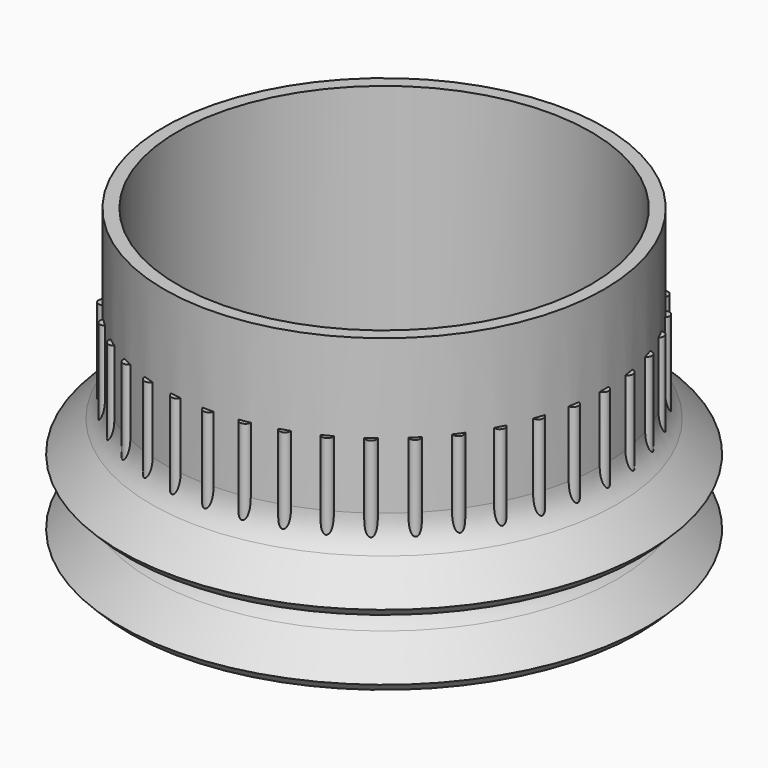
from build123d import *


with BuildPart() as f1:
    # F0 (on Front) → F1 (revolve)
    with BuildSketch(Plane.XZ):
        with BuildLine():
            Line((60, -14.1421356237), (52.9289321881, -7.0710678119))
            ThreePointArc((52.9289321881, -7.0710678119), (50.7612046749, -3.8268343237), (50, 0))
            Line((50, 0), (50, 5.8076118446))
            ThreePointArc((50, 5.8076118446), (50.4038059223, 5.9748737342), (50.8076118446, 5.8076118446))
            Line((50.8076118446, 5.8076118446), (57.8786796564, -1.2634559673))
            Line((57.8786796564, -1.2634559673), (60, 0.8578643763))
            Line((60, 0.8578643763), (52.9289321881, 7.9289321881))
            ThreePointArc((52.9289321881, 7.9289321881), (50.7612046749, 11.1731656763), (50, 15))
            Line((50, 15), (50, 47.5))
            Line((50, 47.5), (50, 50))
            Line((50, 50), (47, 50))
            Line((47, 50), (47, 0))
            ThreePointArc((47, 0), (47.9895660774, -4.9748846207), (50.8076118446, -9.1923881554))
            Line((50.8076118446, -9.1923881554), (57.8786796564, -16.2634559673))
            Line((57.8786796564, -16.2634559673), (60, -14.1421356237))
        make_face()
    revolve(axis=Axis((0, 0, 26.1525176466), (0, 0, 1)))

    # F3 (on offset) → F4 (join, up to the next surface of F1)
    with BuildSketch(Plane.XY.offset(30)):
        with BuildLine():
            ThreePointArc((-1.227725711, 49.9849246231), (0, 50), (1.227725711, 49.9849246231))
            ThreePointArc((1.227725711, 49.9849246231), (0, 51), (-1.227725711, 49.9849246231))
        make_face()
        with BuildLine():
            ThreePointArc((6.6067545733, 49.5615858706), (7.821723252, 49.3844170298), (9.0319753137, 49.177468641))
            ThreePointArc((9.0319753137, 49.177468641), (7.9781577171, 50.3721053704), (6.6067545733, 49.5615858706))
        make_face()
        with BuildLine():
            ThreePointArc((14.2785546334, 47.9178763885), (15.4508497187, 47.5528258148), (16.6138277088, 47.1591001702))
            ThreePointArc((16.6138277088, 47.1591001702), (15.7598667131, 48.5038823311), (14.2785546334, 47.9178763885))
        make_face()
        with BuildLine():
            ThreePointArc((21.5987692907, 45.0942697593), (22.699524987, 44.5503262094), (23.7865925275, 43.9795181412))
            ThreePointArc((23.7865925275, 43.9795181412), (23.1535154867, 45.4413327336), (21.5987692907, 45.0942697593))
        make_face()
        with BuildLine():
            ThreePointArc((28.3871505658, 41.1602925494), (29.3892626146, 40.4508497187), (30.373652495, 39.7170144159))
            ThreePointArc((30.373652495, 39.7170144159), (29.9770478669, 41.2598667131), (28.3871505658, 41.1602925494))
        make_face()
        with BuildLine():
            ThreePointArc((34.4765459824, 36.2128123338), (35.3553390593, 35.3553390593), (36.2128123338, 34.4765459824))
            ThreePointArc((36.2128123338, 34.4765459824), (36.0624458405, 36.0624458405), (34.4765459824, 36.2128123338))
        make_face()
        with BuildLine():
            ThreePointArc((39.7170144159, 30.373652495), (40.4508497187, 29.3892626146), (41.1602925494, 28.3871505658))
            ThreePointArc((41.1602925494, 28.3871505658), (41.2598667131, 29.9770478669), (39.7170144159, 30.373652495))
        make_face()
        with BuildLine():
            ThreePointArc((43.9795181412, 23.7865925275), (44.5503262094, 22.699524987), (45.0942697593, 21.5987692907))
            ThreePointArc((45.0942697593, 21.5987692907), (45.4413327336, 23.1535154867), (43.9795181412, 23.7865925275))
        make_face()
        with BuildLine():
            ThreePointArc((47.1591001702, 16.6138277088), (47.5528258148, 15.4508497187), (47.9178763885, 14.2785546334))
            ThreePointArc((47.9178763885, 14.2785546334), (48.5038823311, 15.7598667131), (47.1591001702, 16.6138277088))
        make_face()
        with BuildLine():
            ThreePointArc((49.177468641, 9.0319753137), (49.3844170298, 7.821723252), (49.5615858706, 6.6067545733))
            ThreePointArc((49.5615858706, 6.6067545733), (50.3721053704, 7.9781577171), (49.177468641, 9.0319753137))
        make_face()
        with BuildLine():
            ThreePointArc((49.9849246231, 1.227725711), (49.9962310137, 0.6139091318), (50, 0))
            ThreePointArc((50, 0), (49.9962310137, -0.6139091318), (49.9849246231, -1.227725711))
            ThreePointArc((49.9849246231, -1.227725711), (51, 0), (49.9849246231, 1.227725711))
        make_face()
        with BuildLine():
            ThreePointArc((49.177468641, -9.0319753137), (50.3721053704, -7.9781577171), (49.5615858706, -6.6067545733))
            ThreePointArc((49.5615858706, -6.6067545733), (49.3844170298, -7.821723252), (49.177468641, -9.0319753137))
        make_face()
        with BuildLine():
            ThreePointArc((47.1591001702, -16.6138277088), (48.5038823311, -15.7598667131), (47.9178763885, -14.2785546334))
            ThreePointArc((47.9178763885, -14.2785546334), (47.5528258148, -15.4508497187), (47.1591001702, -16.6138277088))
        make_face()
        with BuildLine():
            ThreePointArc((43.9795181412, -23.7865925275), (45.4413327336, -23.1535154867), (45.0942697593, -21.5987692907))
            ThreePointArc((45.0942697593, -21.5987692907), (44.5503262094, -22.699524987), (43.9795181412, -23.7865925275))
        make_face()
        with BuildLine():
            ThreePointArc((39.7170144159, -30.373652495), (41.2598667131, -29.9770478669), (41.1602925494, -28.3871505658))
            ThreePointArc((41.1602925494, -28.3871505658), (40.4508497187, -29.3892626146), (39.7170144159, -30.373652495))
        make_face()
        with BuildLine():
            ThreePointArc((34.4765459824, -36.2128123338), (36.0624458405, -36.0624458405), (36.2128123338, -34.4765459824))
            ThreePointArc((36.2128123338, -34.4765459824), (35.3553390593, -35.3553390593), (34.4765459824, -36.2128123338))
        make_face()
        with BuildLine():
            ThreePointArc((28.3871505658, -41.1602925494), (29.9770478669, -41.2598667131), (30.373652495, -39.7170144159))
            ThreePointArc((30.373652495, -39.7170144159), (29.3892626146, -40.4508497187), (28.3871505658, -41.1602925494))
        make_face()
        with BuildLine():
            ThreePointArc((21.5987692907, -45.0942697593), (23.1535154867, -45.4413327336), (23.7865925275, -43.9795181412))
            ThreePointArc((23.7865925275, -43.9795181412), (22.699524987, -44.5503262094), (21.5987692907, -45.0942697593))
        make_face()
        with BuildLine():
            ThreePointArc((14.2785546334, -47.9178763885), (15.7598667131, -48.5038823311), (16.6138277088, -47.1591001702))
            ThreePointArc((16.6138277088, -47.1591001702), (15.4508497187, -47.5528258148), (14.2785546334, -47.9178763885))
        make_face()
        with BuildLine():
            ThreePointArc((6.6067545733, -49.5615858706), (7.9781577171, -50.3721053704), (9.0319753137, -49.177468641))
            ThreePointArc((9.0319753137, -49.177468641), (7.821723252, -49.3844170298), (6.6067545733, -49.5615858706))
        make_face()
        with BuildLine():
            ThreePointArc((-1.227725711, -49.9849246231), (0, -51), (1.227725711, -49.9849246231))
            ThreePointArc((1.227725711, -49.9849246231), (0, -50), (-1.227725711, -49.9849246231))
        make_face()
        with BuildLine():
            ThreePointArc((-9.0319753137, -49.177468641), (-7.9781577171, -50.3721053704), (-6.6067545733, -49.5615858706))
            ThreePointArc((-6.6067545733, -49.5615858706), (-7.821723252, -49.3844170298), (-9.0319753137, -49.177468641))
        make_face()
        with BuildLine():
            ThreePointArc((-16.6138277088, -47.1591001702), (-15.7598667131, -48.5038823311), (-14.2785546334, -47.9178763885))
            ThreePointArc((-14.2785546334, -47.9178763885), (-15.4508497187, -47.5528258148), (-16.6138277088, -47.1591001702))
        make_face()
        with BuildLine():
            ThreePointArc((-23.7865925275, -43.9795181412), (-23.1535154867, -45.4413327336), (-21.5987692907, -45.0942697593))
            ThreePointArc((-21.5987692907, -45.0942697593), (-22.699524987, -44.5503262094), (-23.7865925275, -43.9795181412))
        make_face()
        with BuildLine():
            ThreePointArc((-36.2128123338, -34.4765459824), (-36.0624458405, -36.0624458405), (-34.4765459824, -36.2128123338))
            ThreePointArc((-34.4765459824, -36.2128123338), (-35.3553390593, -35.3553390593), (-36.2128123338, -34.4765459824))
        make_face()
        with BuildLine():
            ThreePointArc((-30.373652495, -39.7170144159), (-29.9770478669, -41.2598667131), (-28.3871505658, -41.1602925494))
            ThreePointArc((-28.3871505658, -41.1602925494), (-29.3892626146, -40.4508497187), (-30.373652495, -39.7170144159))
        make_face()
        with BuildLine():
            ThreePointArc((-41.1602925494, -28.3871505658), (-41.2598667131, -29.9770478669), (-39.7170144159, -30.373652495))
            ThreePointArc((-39.7170144159, -30.373652495), (-40.4508497187, -29.3892626146), (-41.1602925494, -28.3871505658))
        make_face()
        with BuildLine():
            ThreePointArc((-45.0942697593, -21.5987692907), (-45.4413327336, -23.1535154867), (-43.9795181412, -23.7865925275))
            ThreePointArc((-43.9795181412, -23.7865925275), (-44.5503262094, -22.699524987), (-45.0942697593, -21.5987692907))
        make_face()
        with BuildLine():
            ThreePointArc((-47.9178763885, -14.2785546334), (-48.5038823311, -15.7598667131), (-47.1591001702, -16.6138277088))
            ThreePointArc((-47.1591001702, -16.6138277088), (-47.5528258148, -15.4508497187), (-47.9178763885, -14.2785546334))
        make_face()
        with BuildLine():
            ThreePointArc((-49.5615858706, -6.6067545733), (-50.3721053704, -7.9781577171), (-49.177468641, -9.0319753137))
            ThreePointArc((-49.177468641, -9.0319753137), (-49.3844170298, -7.821723252), (-49.5615858706, -6.6067545733))
        make_face()
        with BuildLine():
            ThreePointArc((-49.9849246231, -1.227725711), (-50, 0), (-49.9849246231, 1.227725711))
            ThreePointArc((-49.9849246231, 1.227725711), (-51, 0), (-49.9849246231, -1.227725711))
        make_face()
        with BuildLine():
            ThreePointArc((-49.5615858706, 6.6067545733), (-49.3844170298, 7.821723252), (-49.177468641, 9.0319753137))
            ThreePointArc((-49.177468641, 9.0319753137), (-50.3721053704, 7.9781577171), (-49.5615858706, 6.6067545733))
        make_face()
        with BuildLine():
            ThreePointArc((-47.9178763885, 14.2785546334), (-47.5528258148, 15.4508497187), (-47.1591001702, 16.6138277088))
            ThreePointArc((-47.1591001702, 16.6138277088), (-48.5038823311, 15.7598667131), (-47.9178763885, 14.2785546334))
        make_face()
        with BuildLine():
            ThreePointArc((-45.0942697593, 21.5987692907), (-44.5503262094, 22.699524987), (-43.9795181412, 23.7865925275))
            ThreePointArc((-43.9795181412, 23.7865925275), (-45.4413327336, 23.1535154867), (-45.0942697593, 21.5987692907))
        make_face()
        with BuildLine():
            ThreePointArc((-9.0319753137, 49.177468641), (-7.821723252, 49.3844170298), (-6.6067545733, 49.5615858706))
            ThreePointArc((-6.6067545733, 49.5615858706), (-7.9781577171, 50.3721053704), (-9.0319753137, 49.177468641))
        make_face()
        with BuildLine():
            ThreePointArc((-16.6138277088, 47.1591001702), (-15.4508497187, 47.5528258148), (-14.2785546334, 47.9178763885))
            ThreePointArc((-14.2785546334, 47.9178763885), (-15.7598667131, 48.5038823311), (-16.6138277088, 47.1591001702))
        make_face()
        with BuildLine():
            ThreePointArc((-23.7865925275, 43.9795181412), (-22.699524987, 44.5503262094), (-21.5987692907, 45.0942697593))
            ThreePointArc((-21.5987692907, 45.0942697593), (-23.1535154867, 45.4413327336), (-23.7865925275, 43.9795181412))
        make_face()
        with BuildLine():
            ThreePointArc((-30.373652495, 39.7170144159), (-29.3892626146, 40.4508497187), (-28.3871505658, 41.1602925494))
            ThreePointArc((-28.3871505658, 41.1602925494), (-29.9770478669, 41.2598667131), (-30.373652495, 39.7170144159))
        make_face()
        with BuildLine():
            ThreePointArc((-36.2128123338, 34.4765459824), (-35.3553390593, 35.3553390593), (-34.4765459824, 36.2128123338))
            ThreePointArc((-34.4765459824, 36.2128123338), (-36.0624458405, 36.0624458405), (-36.2128123338, 34.4765459824))
        make_face()
        with BuildLine():
            ThreePointArc((-41.1602925494, 28.3871505658), (-40.4508497187, 29.3892626146), (-39.7170144159, 30.373652495))
            ThreePointArc((-39.7170144159, 30.373652495), (-41.2598667131, 29.9770478669), (-41.1602925494, 28.3871505658))
        make_face()
    extrude(until=Until.NEXT, dir=(0, 0, -1))


solid = f1.part
